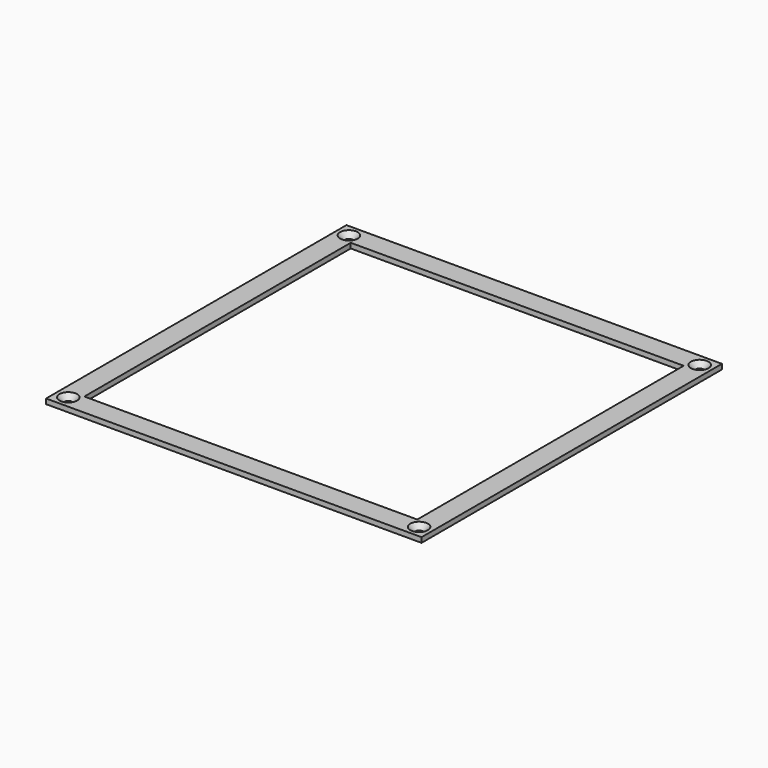
from build123d import *

# Parameters (mm, degrees)
F1_DEPTH  = 5
F0_W      = 115
F0_H      = 3
F0_W_2    = 3
F0_H_2    = 115
F2_DEPTH  = 2
F3_R      = 2.5
F4_DEPTH  = 5
F5_W      = 149
F5_H      = 149
F6_DEPTH  = 35
F7_R      = 1.5
F8_DEPTH  = 35
F9_W      = 149
F9_H      = 50.5775869712
F10_DEPTH = 200
F12_DEPTH = 2
F13_SIZE  = 1.99999


# Not quite as in the source:
# - a fillet or chamfer is up to 0.001 mm smaller than in the source, because OpenCascade refuses the exact size


with BuildPart() as f1:
    # F0 (on Top) → F1 (new body)
    with BuildSketch(Plane.XY):
        Polygon((74.5, 74.5), (60.5, 74.5), (-60.5, 74.5), (-74.5, 74.5), (-74.5, 60.5), (-74.5, -60.5), (-74.5, -74.5), (-60.5, -74.5), (60.5, -74.5), (74.5, -74.5), (74.5, -60.5), (74.5, 60.5), align=None)
        Polygon((57.5, 60.5), (60.5, 60.5), (60.5, 57.5), (60.5, -57.5), (60.5, -60.5), (57.5, -60.5), (-57.5, -60.5), (-60.5, -60.5), (-60.5, -57.5), (-60.5, 57.5), (-60.5, 60.5), (-57.5, 60.5), align=None, mode=Mode.SUBTRACT)
    extrude(amount=F1_DEPTH)

    # F0 (on Top) → F2 (join)
    with BuildSketch(Plane.XY):
        with Locations((0, 59)):
            Rectangle(F0_W, F0_H)
        with Locations((59, 59)):
            Rectangle(F0_W_2, F0_H)
        with Locations((59, 0)):
            Rectangle(F0_W_2, F0_H_2)
        with Locations((59, -59)):
            Rectangle(F0_W_2, F0_H)
        with Locations((0, -59)):
            Rectangle(F0_W, F0_H)
        with Locations((-59, 0)):
            Rectangle(F0_W_2, F0_H_2)
        with Locations((-59, -59)):
            Rectangle(F0_W_2, F0_H)
        with Locations((-59, 59)):
            Rectangle(F0_W_2, F0_H)
    extrude(amount=F2_DEPTH)

    # F3 (on face) → F4 (cut, through all)
    with BuildSketch(Plane.XY.offset(5)):
        with Locations((42.5219088793, 68.0854469538)):
            Circle(F3_R)
    extrude(amount=-F4_DEPTH, mode=Mode.SUBTRACT)

    # F5 (on face) → F6 (join)
    with BuildSketch(Plane.XY.offset(5)):
        Rectangle(F5_W, F5_H)
        Polygon((-60.5, 71.5), (60.5, 71.5), (71.5, 71.5), (71.5, 60.5), (71.5, -60.5), (71.5, -71.5), (60.5, -71.5), (-60.5, -71.5), (-71.5, -71.5), (-71.5, -60.5), (-71.5, 60.5), (-71.5, 71.5), align=None, mode=Mode.SUBTRACT)
    extrude(amount=F6_DEPTH)

    # F7 (on face) → F8 (join)
    with BuildSketch(Plane.XY.offset(40)):
        with BuildLine():
            ThreePointArc((-71.5, 64.975068144), (-66.8161183572, 65.4466893403), (-64.6000009775, 69.6000009775))
            ThreePointArc((-64.6000009775, 69.6000009775), (-64.6946638756, 70.5683335217), (-64.975068144, 71.5))
            Line((-64.975068144, 71.5), (-71.5, 71.5))
            Line((-71.5, 71.5), (-71.5, 64.975068144))
        make_face()
        with Locations((-69.6000009775, 69.6000009775)):
            Circle(F7_R, mode=Mode.SUBTRACT)
        with BuildLine():
            Line((71.5, 71.5), (64.975068144, 71.5))
            ThreePointArc((64.975068144, 71.5), (66.0644670716, 66.0644670716), (71.5, 64.975068144))
            Line((71.5, 64.975068144), (71.5, 71.5))
        make_face()
        with Locations((69.6000009775, 69.6000009775)):
            Circle(F7_R, mode=Mode.SUBTRACT)
        with BuildLine():
            Line((71.5, -71.5), (71.5, -64.975068144))
            ThreePointArc((71.5, -64.975068144), (66.0644670716, -66.0644670716), (64.975068144, -71.5))
            Line((64.975068144, -71.5), (71.5, -71.5))
        make_face()
        with Locations((69.6000009775, -69.6000009775)):
            Circle(F7_R, mode=Mode.SUBTRACT)
        with BuildLine():
            ThreePointArc((-64.6000009775, -69.6000009775), (-66.8161183572, -65.4466893403), (-71.5, -64.975068144))
            Line((-71.5, -64.975068144), (-71.5, -71.5))
            Line((-71.5, -71.5), (-64.975068144, -71.5))
            ThreePointArc((-64.975068144, -71.5), (-64.6946638756, -70.5683335217), (-64.6000009775, -69.6000009775))
        make_face()
        with Locations((-69.6000009775, -69.6000009775)):
            Circle(F7_R, mode=Mode.SUBTRACT)
    extrude(amount=-F8_DEPTH)

    # F9 (on face) → F10 (cut)
    with BuildSketch(Plane.XZ.offset(74.5)):
        with Locations((0, 12.7112065144)):
            Rectangle(F9_W, F9_H)
    extrude(amount=-F10_DEPTH, mode=Mode.SUBTRACT)

    # F11 (on face) → F12 (join)
    with BuildSketch(Plane.XY.offset(40)):
        with BuildLine():
            ThreePointArc((-64.975068144, 71.5), (-64.6974956073, 68.6174323567), (-66.0644670716, 66.0644670716))
            Line((-66.0644670716, 66.0644670716), (66.0644670716, 66.0644670716))
            ThreePointArc((66.0644670716, 66.0644670716), (64.6974956073, 68.6174323567), (64.975068144, 71.5))
            Line((64.975068144, 71.5), (-64.975068144, 71.5))
        make_face()
        with BuildLine():
            ThreePointArc((71.5, 64.975068144), (68.6174323567, 64.6974956073), (66.0644670716, 66.0644670716))
            Line((66.0644670716, 66.0644670716), (66.0644670716, -66.0644670716))
            ThreePointArc((66.0644670716, -66.0644670716), (68.6174323567, -64.6974956073), (71.5, -64.975068144))
            Line((71.5, -64.975068144), (71.5, 64.975068144))
        make_face()
        with BuildLine():
            Line((66.0644670716, -66.0644670716), (-66.0644670716, -66.0644670716))
            ThreePointArc((-66.0644670716, -66.0644670716), (-64.6974956073, -68.6174323567), (-64.975068144, -71.5))
            Line((-64.975068144, -71.5), (64.975068144, -71.5))
            ThreePointArc((64.975068144, -71.5), (64.6974956073, -68.6174323567), (66.0644670716, -66.0644670716))
        make_face()
        with BuildLine():
            Line((-66.0644670716, -66.0644670716), (-66.0644670716, 66.0644670716))
            ThreePointArc((-66.0644670716, 66.0644670716), (-68.6174323567, 64.6974956073), (-71.5, 64.975068144))
            Line((-71.5, 64.975068144), (-71.5, -64.975068144))
            ThreePointArc((-71.5, -64.975068144), (-68.6174323567, -64.6974956073), (-66.0644670716, -66.0644670716))
        make_face()
    extrude(amount=-F12_DEPTH)

    # F13 (size 2 in the source; OpenCascade refuses exactly that, so slightly less here)
    f13_edges = [f1.edges().sort_by_distance(p)[0] for p in [
        (-71.100001, 69.600001, 40),
        (68.100001, 69.600001, 40),
        (68.100001, -69.600001, 40),
        (-71.100001, -69.600001, 40),
    ]]
    chamfer(f13_edges, length=F13_SIZE)


solid = f1.part
